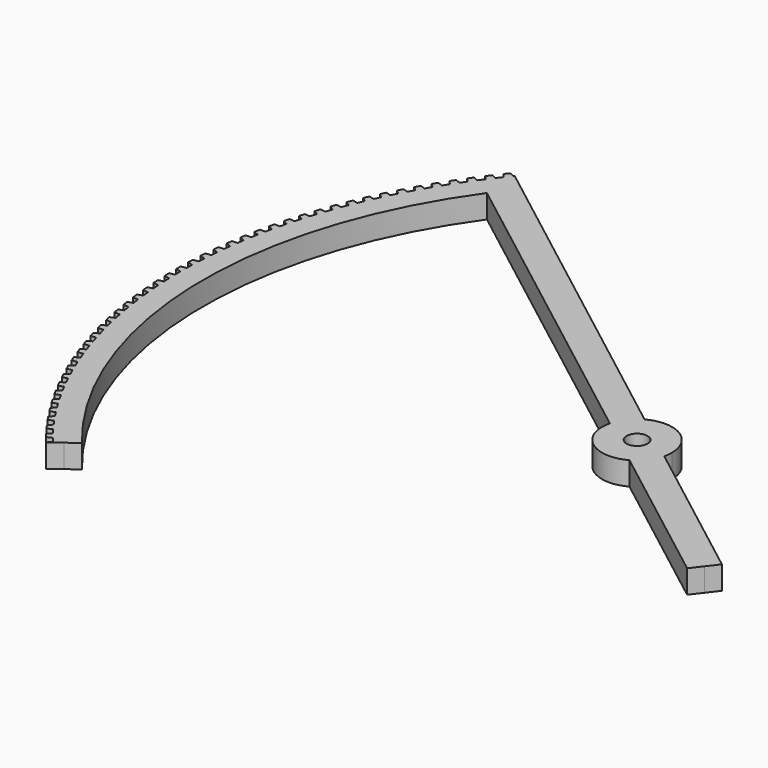
from build123d import *

# Parameters (mm, degrees)
F1_DEPTH         = 10
F3_DEPTH         = 10
F4_R             = 4.5
F5_DEPTH         = 10.001
F7_DEPTH         = 25
F7_COPIES_COUNT  = 43
F7_COPIES_ANGLE  = 76.3636363636
F7_COPIES1_COUNT = 2
F7_COPIES1_ANGLE = 358.1818


# Not quite as in the source:
# - a pattern or mirror of a feature is missing from the dataset's text; its kind, count and spacing are read off the source's solid


with BuildPart() as f1:
    # F0 (on Top) → F1 (new body)
    with BuildSketch(Plane.XY):
        with BuildLine():
            Line((-152.3238413359, 116.8821943697), (75, -57.5495240984))
            Line((75, -57.5495240984), (78.6525685741, -52.7894040567))
            Line((78.6525685741, -52.7894040567), (-153.3592532079, 125.2395283268))
            ThreePointArc((-153.3592532079, 125.2395283268), (-198, 0), (-153.3592532079, -125.2395283268))
            Line((-153.3592532079, -125.2395283268), (-148.5968777189, -121.5852290872))
            ThreePointArc((-148.5968777189, -121.5852290872), (-191.9765553438, -3.0003663675), (-152.3238413359, 116.8821943697))
        make_face()
        with BuildLine():
            Line((71.3474314259, -62.3096441402), (75, -57.5495240984))
            Line((75, -57.5495240984), (-152.3238413359, 116.8821943697))
            ThreePointArc((-152.3238413359, 116.8821943697), (-191.9765553438, -3.0003663675), (-148.5968777189, -121.5852290872))
            Line((-148.5968777189, -121.5852290872), (-143.834356607, -117.9308181072))
            ThreePointArc((-143.834356607, -117.9308181072), (-185.903200618, -6), (-151.1394937551, 108.4105780237))
            Line((-151.1394937551, 108.4105780237), (71.3474314259, -62.3096441402))
        make_face()
    extrude(amount=F1_DEPTH)

    # F2 (on face) → F3 (join)
    with BuildSketch(Plane.XY.offset(10)):
        with BuildLine():
            ThreePointArc((14.5593737782, -3.6089659441), (14.8894359644, -1.8178824668), (15, 0))
            ThreePointArc((15, 0), (7.6218911875, 12.9192404856), (-7.2542366301, 13.1292060276))
            Line((-7.2542366301, 13.1292060276), (14.5593737782, -3.6089659441))
        make_face()
        with BuildLine():
            Line((14.5593737782, -3.6089659441), (-7.2542366301, 13.1292060276))
            ThreePointArc((-7.2542366301, 13.1292060276), (-11.9003001044, 9.1314214351), (-14.5593737782, 3.6089659441))
            Line((-14.5593737782, 3.6089659441), (7.2542366301, -13.1292060276))
            ThreePointArc((7.2542366301, -13.1292060276), (11.9003001044, -9.1314214351), (14.5593737782, -3.6089659441))
        make_face()
        with BuildLine():
            Line((7.2542366301, -13.1292060276), (-14.5593737782, 3.6089659441))
            ThreePointArc((-14.5593737782, 3.6089659441), (-9.1314214351, -11.9003001044), (7.2542366301, -13.1292060276))
        make_face()
    extrude(amount=-F3_DEPTH)

    # F4 (on face) → F5 (cut, through all)
    with BuildSketch(Plane.XY.offset(10)):
        Circle(F4_R)
    extrude(amount=-F5_DEPTH, mode=Mode.SUBTRACT)

    # F6 (on face) → F7 (cut)
    with BuildSketch(Plane.XY.offset(10)):
        with BuildLine():
            ThreePointArc((-155.7425092251, 118.5847094708), (-154.8713533719, 119.7202004874), (-153.9919190308, 120.8492919847))
            Line((-153.9919190308, 120.8492919847), (-155.4369141598, 122.6513991624))
            ThreePointArc((-155.4369141598, 122.6513991624), (-156.6267371711, 121.1283005871), (-157.8016361839, 119.593660441))
            Line((-157.8016361839, 119.593660441), (-155.7425092251, 118.5847094707))
        make_face()
    f7 = extrude(amount=-F7_DEPTH, mode=Mode.SUBTRACT)

    # F7_copies: F7 ×43 about axis
    f7_copies_axis = Axis((0, 0, 0), (0, 0, 1))
    for i in range(1, F7_COPIES_COUNT):
        add(f7.rotate(f7_copies_axis, i * F7_COPIES_ANGLE / (F7_COPIES_COUNT - 1)), mode=Mode.SUBTRACT)

    # F7_copies1: F7 ×2 about axis
    f7_copies1_axis = Axis((0, 0, 0), (0, 0, 1))
    for i in range(1, F7_COPIES1_COUNT):
        add(f7.rotate(f7_copies1_axis, i * F7_COPIES1_ANGLE / (F7_COPIES1_COUNT - 1)), mode=Mode.SUBTRACT)


solid = f1.part
